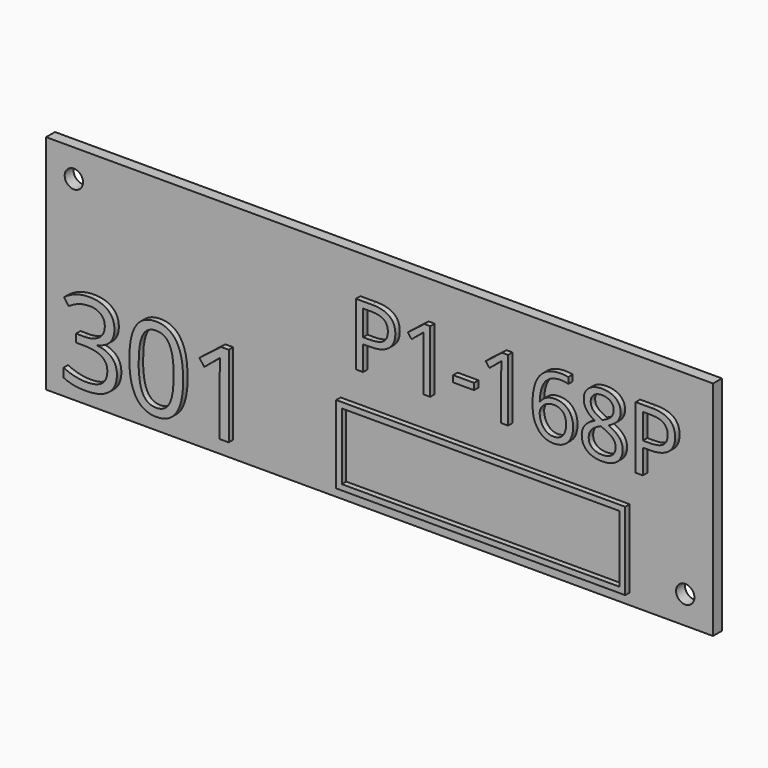
from build123d import *

# Parameters (mm, degrees)
F0_W         = 120
F0_H         = 40
F1_DEPTH     = 2
F3_D         = 3.3
F4_TEXT_SIZE = 15.681149951
F5_DEPTH     = 1
F6_TEXT_SIZE = 20.5478077656
F7_DEPTH     = 1
F8_W         = 52
F8_H         = 14
F8_W_2       = 49.99999962
F8_H_2       = 11.99999962
F9_DEPTH     = 1


# Not quite as in the source:
# - Text() gives the source's letters only with a copy of the font that has no kerning and outlines rounded to 1/6400 em; it was checked with that copy


with BuildPart() as f1:
    # F0 (on Front) → F1 (new body)
    with BuildSketch(Plane.XZ):
        Rectangle(F0_W, F0_H)
    extrude(amount=F1_DEPTH)

    # F3 (through all)
    with Locations(Plane.XZ.offset(2)):
        with Locations((-55, 15), (55, -15)):
            Hole(F3_D / 2)

    # F4 (on face) → F5 (join)
    with BuildSketch(Plane.XZ.offset(2)):
        with Locations((-5, 2)):
            Text('P1-168P', F4_TEXT_SIZE, font='Open Sans', text_align=(TextAlign.LEFT, TextAlign.BOTTOM))
    extrude(amount=F5_DEPTH)

    # F6 (on face) → F7 (join)
    with BuildSketch(Plane.XZ.offset(2)):
        with Locations((-57, -17)):
            Text('301', F6_TEXT_SIZE, font='Open Sans', text_align=(TextAlign.LEFT, TextAlign.BOTTOM))
    extrude(amount=F7_DEPTH)

    # F8 (on face) → F9 (join)
    with BuildSketch(Plane.XZ.offset(2)):
        with Locations((19, -11)):
            Rectangle(F8_W, F8_H)
        with Locations((19, -11)):
            Rectangle(F8_W_2, F8_H_2, mode=Mode.SUBTRACT)
    extrude(amount=F9_DEPTH)


solid = f1.part
